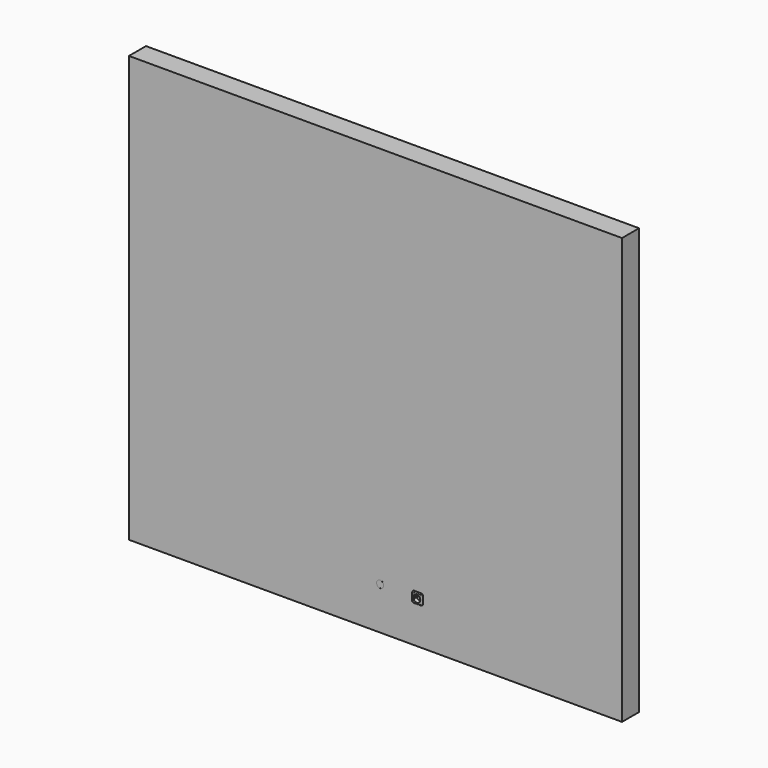
from build123d import *

# Parameters (mm, degrees)
F0_W         = 3472.3631921678
F0_H         = 3000
F1_DEPTH     = 150
F2_R         = 25
F2_R_2       = 24.95
F3_DEPTH     = 50
F4_W         = 74.9007655587
F4_H         = 74.9007655587
F5_DEPTH     = 8
F6_R         = 13
F7_T1_DEPTH  = 48.9007655587
F7_T3_DEPTH  = 48.9007655587
F7_T6_ANGLE  = 90
F7_T8_ANGLE  = 90
F7_T10_ANGLE = 90
F7_T12_ANGLE = 90
F4_R         = 2.6271162968
F8_DEPTH     = 20
F9_DEPTH     = 40


# Not quite as in the source:
# - a fillet or chamfer that OpenCascade refuses, or shapes differently, is made with other operations: its cross-section is extruded or revolved along the edge and cut away or added


with BuildPart() as f1:
    # F0 (on Front) → F1 (new body)
    with BuildSketch(Plane.XZ):
        with Locations((1736.1815960839, 1500)):
            Rectangle(F0_W, F0_H)
    extrude(amount=F1_DEPTH)

    # F2 (on face) → F3 (cut)
    with BuildSketch(Plane.XZ.offset(150)):
        with Locations((1768.8783407211, 300)):
            Circle(F2_R)
        with Locations((1768.8783407211, 300)):
            Circle(F2_R_2, mode=Mode.SUBTRACT)
    extrude(amount=-F3_DEPTH, mode=Mode.SUBTRACT)

    # F4 (on face) → F5 (join)
    with BuildSketch(Plane.XZ.offset(150)):
        with Locations((2033.8273048401, 300)):
            Rectangle(F4_W, F4_H)
        with BuildLine():
            ThreePointArc((2056.8177885488, 290.179732242), (2033.8273048401, 275), (2010.8368211313, 290.179732242))
            Line((2010.8368211313, 290.179732242), (2010.8368211313, 297.4973082542))
            Line((2010.8368211313, 297.4973082542), (2008.9528895902, 297.4973082542))
            Line((2008.9528895902, 297.4973082542), (2008.9528895902, 302.5026917458))
            Line((2008.9528895902, 302.5026917458), (2010.8368211313, 302.5026917458))
            Line((2010.8368211313, 302.5026917458), (2010.8368211313, 309.820267758))
            ThreePointArc((2010.8368211313, 309.820267758), (2020.0524490141, 320.8627262594), (2033.8273048401, 325))
            ThreePointArc((2033.8273048401, 325), (2047.602160666, 320.8627262594), (2056.8177885488, 309.820267758))
            Line((2056.8177885488, 309.820267758), (2056.8177885488, 302.5026917458))
            Line((2056.8177885488, 302.5026917458), (2058.70172009, 302.5026917458))
            Line((2058.70172009, 302.5026917458), (2058.70172009, 297.4973082542))
            Line((2058.70172009, 297.4973082542), (2056.8177885488, 297.4973082542))
            Line((2056.8177885488, 297.4973082542), (2056.8177885488, 290.179732242))
        make_face(mode=Mode.SUBTRACT)
    extrude(amount=F5_DEPTH)

    # F6
    f6_edges = [f1.edges().sort_by_distance(p)[0] for p in [
        (1996.376922, -154, 337.450383),
        (1996.376922, -154, 262.549617),
        (2071.277688, -154, 262.549617),
        (2071.277688, -154, 337.450383),
    ]]
    fillet(f6_edges, radius=F6_R)

    # F7: fillet of radius 6.7597979746 on 8 edges, made by hand

    # F7_s2 → F7_t1 (cut)
    with BuildSketch(Plane.YZ.offset(2009.3769220608)):
        with BuildLine():
            add(Edge.make_bspline(
                [(-151.2402020254, 337.4503827793), (-158, 337.4503827793), (-158, 330.6905848047)],
                knots=[0, 0, 0, 1, 1, 1], degree=2, weights=[1, 0.4285714286, 1]))
            Line((-158, 330.6905848047), (-158, 337.4503827793))
            Line((-158, 337.4503827793), (-151.2402020254, 337.4503827793))
        make_face()
        with BuildLine():
            add(Edge.make_bspline(
                [(-151.2402020254, 262.5496172207), (-158, 262.5496172207), (-158, 269.3094151953)],
                knots=[0, 0, 0, 1, 1, 1], degree=2, weights=[1, 0.4285714286, 1]))
            Line((-158, 269.3094151953), (-158, 262.5496172207))
            Line((-158, 262.5496172207), (-151.2402020254, 262.5496172207))
        make_face()
    extrude(amount=F7_T1_DEPTH, mode=Mode.SUBTRACT)

    # F7_s4 → F7_t3 (cut)
    with BuildSketch(Plane.XY.offset(275.5496172207)):
        with BuildLine():
            add(Edge.make_bspline(
                [(2071.2776876194, -151.2402020254), (2071.2776876194, -158), (2064.5178896448, -158)],
                knots=[0, 0, 0, 1, 1, 1], degree=2, weights=[1, 0.4285714286, 1]))
            Line((2064.5178896448, -158), (2071.2776876194, -158))
            Line((2071.2776876194, -158), (2071.2776876194, -151.2402020254))
        make_face()
        with BuildLine():
            add(Edge.make_bspline(
                [(1996.3769220608, -151.2402020254), (1996.3769220608, -158), (2003.1367200354, -158)],
                knots=[0, 0, 0, 1, 1, 1], degree=2, weights=[1, 0.4285714286, 1]))
            Line((2003.1367200354, -158), (1996.3769220608, -158))
            Line((1996.3769220608, -158), (1996.3769220608, -151.2402020254))
        make_face()
    extrude(amount=F7_T3_DEPTH, mode=Mode.SUBTRACT)

    # F7_s5 → F7_t6 (revolve, cut)
    with BuildSketch(Plane.YZ.offset(2009.3769220608)):
        with BuildLine():
            add(Edge.make_bspline(
                [(-151.2402020254, 337.4503827793), (-158, 337.4503827793), (-158, 330.6905848047)],
                knots=[0, 0, 0, 1, 1, 1], degree=2, weights=[1, 0.4285714286, 1]))
            Line((-158, 330.6905848047), (-158, 337.4503827793))
            Line((-158, 337.4503827793), (-151.2402020254, 337.4503827793))
        make_face()
    revolve(axis=Axis((2009.3769220608, -158, 324.4503827793), (0, -1, 0)), revolution_arc=F7_T6_ANGLE, mode=Mode.SUBTRACT)

    # F7_s7 → F7_t8 (revolve, cut)
    with BuildSketch(Plane.XY.offset(324.4503827793)):
        with BuildLine():
            add(Edge.make_bspline(
                [(2071.2776876194, -151.2402020254), (2071.2776876194, -158), (2064.5178896448, -158)],
                knots=[0, 0, 0, 1, 1, 1], degree=2, weights=[1, 0.4285714286, 1]))
            Line((2064.5178896448, -158), (2071.2776876194, -158))
            Line((2071.2776876194, -158), (2071.2776876194, -151.2402020254))
        make_face()
    revolve(axis=Axis((2058.2776876194, -158, 324.4503827793), (0, -1, 0)), revolution_arc=F7_T8_ANGLE, mode=Mode.SUBTRACT)

    # F7_s9 → F7_t10 (revolve, cut)
    with BuildSketch(Plane.XY.offset(275.5496172207)):
        with BuildLine():
            add(Edge.make_bspline(
                [(2071.2776876194, -151.2402020254), (2071.2776876194, -158), (2064.5178896448, -158)],
                knots=[0, 0, 0, 1, 1, 1], degree=2, weights=[1, 0.4285714286, 1]))
            Line((2064.5178896448, -158), (2071.2776876194, -158))
            Line((2071.2776876194, -158), (2071.2776876194, -151.2402020254))
        make_face()
    revolve(axis=Axis((2058.2776876194, -158, 275.5496172207), (0, 1, 0)), revolution_arc=F7_T10_ANGLE, mode=Mode.SUBTRACT)

    # F7_s11 → F7_t12 (revolve, cut)
    with BuildSketch(Plane.XY.offset(275.5496172207)):
        with BuildLine():
            add(Edge.make_bspline(
                [(1996.3769220608, -151.2402020254), (1996.3769220608, -158), (2003.1367200354, -158)],
                knots=[0, 0, 0, 1, 1, 1], degree=2, weights=[1, 0.4285714286, 1]))
            Line((2003.1367200354, -158), (1996.3769220608, -158))
            Line((1996.3769220608, -158), (1996.3769220608, -151.2402020254))
        make_face()
    revolve(axis=Axis((2009.3769220608, -158, 275.5496172207), (0, -1, 0)), revolution_arc=F7_T12_ANGLE, mode=Mode.SUBTRACT)

    # F4 (on face) → F8 (cut)
    with BuildSketch(Plane.XZ.offset(150)):
        with BuildLine():
            Line((2010.8368211313, 297.4973082542), (2010.8368211313, 290.179732242))
            ThreePointArc((2010.8368211313, 290.179732242), (2033.8273048401, 275), (2056.8177885488, 290.179732242))
            Line((2056.8177885488, 290.179732242), (2056.8177885488, 297.4973082542))
            Line((2056.8177885488, 297.4973082542), (2058.70172009, 297.4973082542))
            Line((2058.70172009, 297.4973082542), (2058.70172009, 302.5026917458))
            Line((2058.70172009, 302.5026917458), (2056.8177885488, 302.5026917458))
            Line((2056.8177885488, 302.5026917458), (2056.8177885488, 309.820267758))
            ThreePointArc((2056.8177885488, 309.820267758), (2047.602160666, 320.8627262594), (2033.8273048401, 325))
            ThreePointArc((2033.8273048401, 325), (2020.0524490141, 320.8627262594), (2010.8368211313, 309.820267758))
            Line((2010.8368211313, 309.820267758), (2010.8368211313, 302.5026917458))
            Line((2010.8368211313, 302.5026917458), (2008.9528895902, 302.5026917458))
            Line((2008.9528895902, 302.5026917458), (2008.9528895902, 297.4973082542))
            Line((2008.9528895902, 297.4973082542), (2010.8368211313, 297.4973082542))
        make_face()
        with Locations((2022.7699279785, 300)):
            Circle(F4_R, mode=Mode.SUBTRACT)
        with Locations((2044.8846817017, 300)):
            Circle(F4_R, mode=Mode.SUBTRACT)
    extrude(amount=-F8_DEPTH, mode=Mode.SUBTRACT)

    # F9 (cut): faces of the model
    f9_faces = [f1.faces().sort_by_distance(p)[0] for p in [
        (2022.7699279785, -150, 300),
        (2044.8846817017, -150, 300),
    ]]
    extrude(f9_faces, amount=-F9_DEPTH, mode=Mode.SUBTRACT)


solid = f1.part
